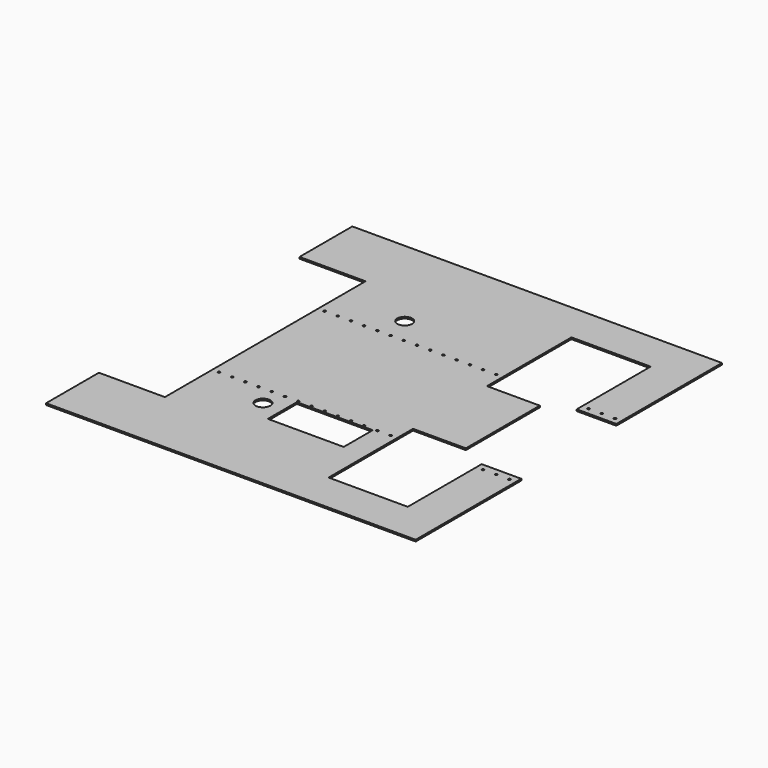
from build123d import *

# Parameters (mm, degrees)
F0_R     = 2.1844
F0_R_2   = 14.2875
F0_W     = 50.8
F0_H     = 177.8
F0_W_2   = 196.85
F0_H_2   = 9.525
F1_DEPTH = 3.175


# Not quite as in the source:
# - a feature names something its author has since deleted; it is built from what else it names


with BuildPart() as f1:
    # F0 (on Top) → F1 (new body)
    with BuildSketch(Plane.XY):
        Polygon((431.8, 0), (0, 0), (0, -127), (127, -127), (127, -609.6), (0, -609.6), (0, -736.6), (431.8, -736.6), (431.8, -660.4), (482.6, -660.4), (482.6, -457.2), (584.2, -457.2), (584.2, -366.7125), (387.35, -366.7125), (387.35, -357.1875), (584.2, -357.1875), (584.2, -279.4), (482.6, -279.4), (482.6, -76.2), (431.8, -76.2), align=None)
        with Locations((139.7, -495.3)):
            Circle(F0_R, mode=Mode.SUBTRACT)
        with Locations((165.1, -495.3)):
            Circle(F0_R, mode=Mode.SUBTRACT)
        with Locations((254, -532.4475)):
            Circle(F0_R_2, mode=Mode.SUBTRACT)
        with Locations((190.5, -495.3)):
            Circle(F0_R, mode=Mode.SUBTRACT)
        with Locations((215.9, -495.3)):
            Circle(F0_R, mode=Mode.SUBTRACT)
        with Locations((241.3, -495.3)):
            Circle(F0_R, mode=Mode.SUBTRACT)
        with Locations((266.7, -495.3)):
            Circle(F0_R, mode=Mode.SUBTRACT)
        with Locations((292.1, -495.3)):
            Circle(F0_R, mode=Mode.SUBTRACT)
        with Locations((317.5, -495.3)):
            Circle(F0_R, mode=Mode.SUBTRACT)
        with Locations((342.9, -495.3)):
            Circle(F0_R, mode=Mode.SUBTRACT)
        Polygon((387.35, -498.475), (438.15, -498.475), (438.15, -568.325), (292.1, -568.325), (292.1, -498.475), align=None, mode=Mode.SUBTRACT)
        with Locations((368.3, -495.3)):
            Circle(F0_R, mode=Mode.SUBTRACT)
        with Locations((393.7, -495.3)):
            Circle(F0_R, mode=Mode.SUBTRACT)
        with Locations((419.1, -495.3)):
            Circle(F0_R, mode=Mode.SUBTRACT)
        with Locations((444.5, -495.3)):
            Circle(F0_R, mode=Mode.SUBTRACT)
        with Locations((469.9, -495.3)):
            Circle(F0_R, mode=Mode.SUBTRACT)
        with Locations((139.7, -241.3)):
            Circle(F0_R, mode=Mode.SUBTRACT)
        with Locations((165.1, -241.3)):
            Circle(F0_R, mode=Mode.SUBTRACT)
        with Locations((190.5, -241.3)):
            Circle(F0_R, mode=Mode.SUBTRACT)
        with Locations((215.9, -241.3)):
            Circle(F0_R, mode=Mode.SUBTRACT)
        with Locations((241.3, -241.3)):
            Circle(F0_R, mode=Mode.SUBTRACT)
        with Locations((266.7, -241.3)):
            Circle(F0_R, mode=Mode.SUBTRACT)
        with Locations((254, -191.4525)):
            Circle(F0_R_2, mode=Mode.SUBTRACT)
        with Locations((292.1, -241.3)):
            Circle(F0_R, mode=Mode.SUBTRACT)
        with Locations((317.5, -241.3)):
            Circle(F0_R, mode=Mode.SUBTRACT)
        with Locations((342.9, -241.3)):
            Circle(F0_R, mode=Mode.SUBTRACT)
        with Locations((368.3, -241.3)):
            Circle(F0_R, mode=Mode.SUBTRACT)
        with Locations((393.7, -241.3)):
            Circle(F0_R, mode=Mode.SUBTRACT)
        with Locations((419.1, -241.3)):
            Circle(F0_R, mode=Mode.SUBTRACT)
        with Locations((444.5, -241.3)):
            Circle(F0_R, mode=Mode.SUBTRACT)
        with Locations((469.9, -241.3)):
            Circle(F0_R, mode=Mode.SUBTRACT)
        Polygon((685.8, 0), (431.8, 0), (431.8, -76.2), (482.6, -76.2), (635, -76.2), (685.8, -76.2), align=None)
        Polygon((711.2, 0), (685.8, 0), (685.8, -76.2), (685.8, -254), (711.2, -254), align=None)
        with Locations((698.5, -241.3)):
            Circle(F0_R, mode=Mode.SUBTRACT)
        with Locations((660.4, -165.1)):
            Rectangle(F0_W, F0_H)
        with Locations((647.7, -241.3)):
            Circle(F0_R, mode=Mode.SUBTRACT)
        with Locations((673.1, -241.3)):
            Circle(F0_R, mode=Mode.SUBTRACT)
        Polygon((431.8, -660.4), (431.8, -736.6), (685.8, -736.6), (685.8, -660.4), (635, -660.4), (482.6, -660.4), align=None)
        Polygon((711.2, -736.6), (711.2, -482.6), (685.8, -482.6), (685.8, -660.4), (685.8, -736.6), align=None)
        with Locations((698.5, -495.3)):
            Circle(F0_R, mode=Mode.SUBTRACT)
        with Locations((660.4, -571.5)):
            Rectangle(F0_W, F0_H)
        with Locations((647.7, -495.3)):
            Circle(F0_R, mode=Mode.SUBTRACT)
        with Locations((673.1, -495.3)):
            Circle(F0_R, mode=Mode.SUBTRACT)
        with Locations((485.775, -361.95)):
            Rectangle(F0_W_2, F0_H_2)
    extrude(amount=F1_DEPTH)


solid = f1.part
